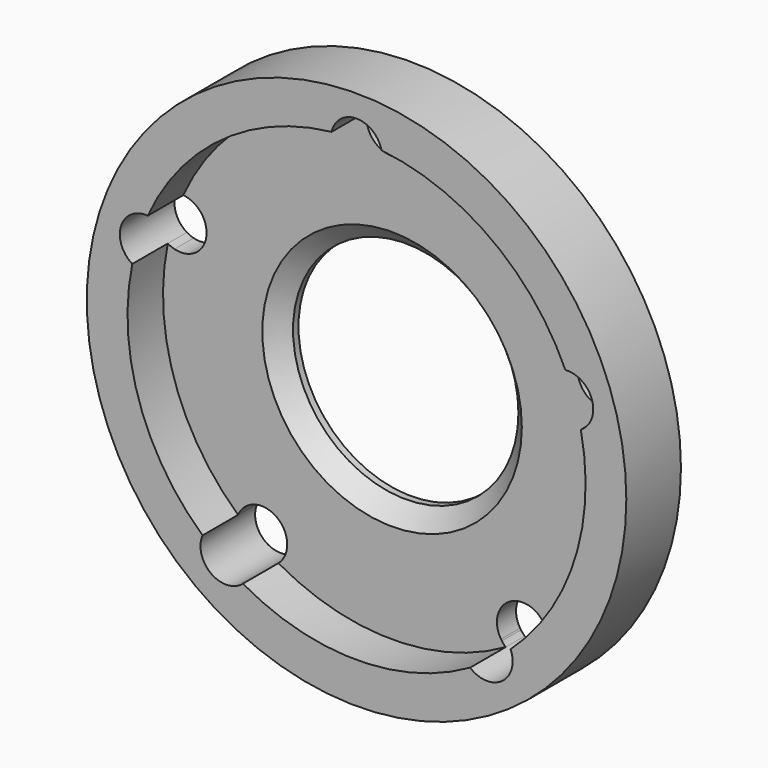
from build123d import *

# Parameters (mm, degrees)
F0_R            = 79
F0_R_2          = 33
F1_DEPTH        = 20
F2_R            = 67.075
F3_DEPTH        = 13
F4_SIZE         = 5
F6_DEPTH        = 20.001
F6_COPIES_COUNT = 5


# Not quite as in the source:
# - a pattern or mirror of a feature is missing from the dataset's text; its kind, count and spacing are read off the source's solid


with BuildPart() as f1:
    # F0 (on Front) → F1 (new body)
    with BuildSketch(Plane.XZ):
        Circle(F0_R)
        Circle(F0_R_2, mode=Mode.SUBTRACT)
    extrude(amount=F1_DEPTH)

    # F2 (on face) → F3 (cut)
    with BuildSketch(Plane.XZ.offset(20)):
        Circle(F2_R)
    extrude(amount=-F3_DEPTH, mode=Mode.SUBTRACT)

    # F4
    f4_edges = [f1.edges().sort_by_distance(p)[0] for p in [
        (-33, -7, 0),
    ]]
    chamfer(f4_edges, length=F4_SIZE)

    # F5 (on face) → F6 (cut, through all)
    with BuildSketch(Plane.XZ.offset(20)):
        with BuildLine():
            ThreePointArc((-7.4875080879, 64.5673076923), (0, 57.5), (7.4875080879, 64.5673076923))
            ThreePointArc((7.4875080879, 64.5673076923), (0, 65), (-7.4875080879, 64.5673076923))
        make_face()
        with BuildLine():
            ThreePointArc((-7.4875080879, 64.5673076923), (0, 65), (7.4875080879, 64.5673076923))
            ThreePointArc((7.4875080879, 64.5673076923), (7.4968763715, 64.7835637039), (7.5, 65))
            ThreePointArc((7.5, 65), (7.4524663535, 65.843057086), (7.3104679333, 66.6754278846))
            ThreePointArc((7.3104679333, 66.6754278846), (0, 67.075), (-7.3104679333, 66.6754278846))
            ThreePointArc((-7.3104679333, 66.6754278846), (-7.4736916091, 65.6276414045), (-7.4875080879, 64.5673076923))
        make_face()
        with BuildLine():
            ThreePointArc((7.3104679333, 66.6754278846), (0, 72.5), (-7.3104679333, 66.6754278846))
            ThreePointArc((-7.3104679333, 66.6754278846), (0, 67.075), (7.3104679333, 66.6754278846))
        make_face()
    f6 = extrude(amount=-F6_DEPTH, mode=Mode.SUBTRACT)

    # F6_copies: F6 ×5 about axis
    f6_copies_axis = Axis((0, 0, 0), (0, 1, 0))
    for i in range(1, F6_COPIES_COUNT):
        add(f6.rotate(f6_copies_axis, i * 360 / F6_COPIES_COUNT), mode=Mode.SUBTRACT)


solid = f1.part
